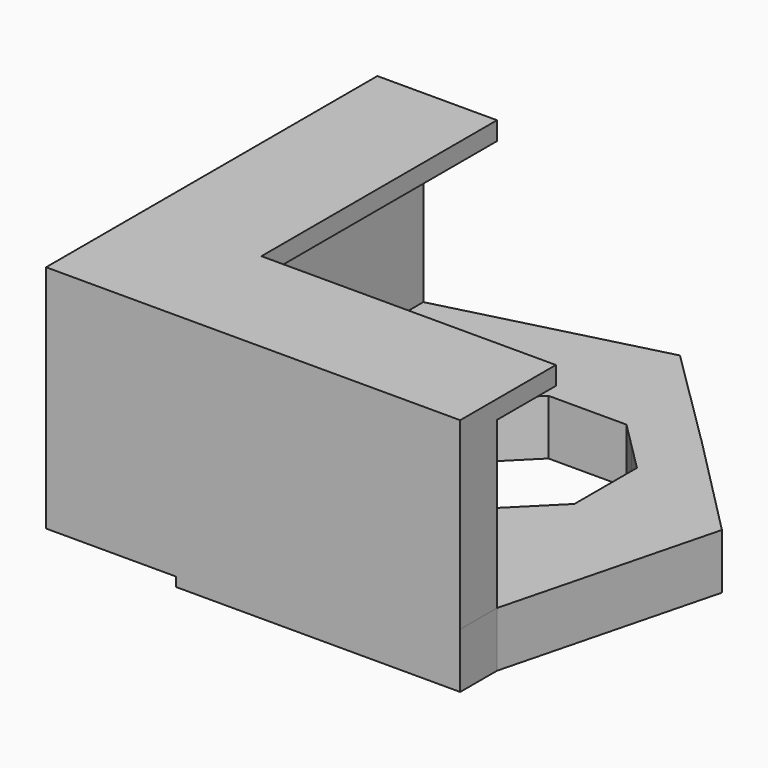
from build123d import *

# Parameters (mm, degrees)
F2_DEPTH  = 6
F4_DEPTH  = 3
F5_DEPTH  = 6.5
F7_DEPTH  = 1.5
F8_R      = 0.99999
F10_DEPTH = 1


# Not quite as in the source:
# - a fillet or chamfer is up to 0.001 mm smaller than in the source, because OpenCascade refuses the exact size


with BuildPart() as f2:
    # F1 (on offset) → F2 (new body)
    with BuildSketch(Plane.XY.offset(4)):
        Polygon((20, 0), (0, 0), (0, 20), (-2.5, 20), (-2.5, -2.5), (20, -2.5), align=None)
    extrude(amount=F2_DEPTH)



with BuildPart() as f4:
    # F3 (on Top) → F4 (new body)
    with BuildSketch(Plane.XY):
        Polygon((16.591883092, 13.7634559673), (16.591883092, 9.5208152802), (4.5710678119, -2.5), (8.75, -2.5), (22.9713253162, 11.5625), (17.2989898732, 17.2989898732), (15.1776695297, 15.1776695297), align=None)
        Polygon((22.9713253162, 11.5625), (8.75, -2.5), (20, -2.5), (20.0004931539, 0), align=None)
        Polygon((13.7634559673, 16.591883092), (15.1776695297, 15.1776695297), (17.2989898732, 17.2989898732), (11.5625, 22.9713253162), (-2.5, 8.75), (-2.5, 4.5710678119), (9.5208152802, 16.591883092), align=None)
        Polygon((-2.5, 8.75), (11.5625, 22.9713253162), (0, 19.9992582202), (-2.5, 20), align=None)
    extrude(amount=-F4_DEPTH)


with BuildPart() as f2_1:
    add(f2.part)

    add(f4.part)  # F5 merges F4
    # F1 (on offset) → F5 (join)
    with BuildSketch(Plane.XY.offset(4)):
        Polygon((20, 0), (0, 0), (0, 20), (-2.5, 20), (-2.5, -2.5), (20, -2.5), align=None)
    extrude(amount=-F5_DEPTH)

    # F6 (on face) → F7 (join)
    with BuildSketch(Plane(origin=(15.1776695297, 15.1776695297, 0), x_dir=(0.7071067812, -0.7071067812, 0), z_dir=(-0.7071067812, -0.7071067812, 0))):
        with BuildLine():
            Line((-1, -3), (1, -3))
            ThreePointArc((1, -3), (0, -2), (-1, -3))
        make_face()
    extrude(amount=F7_DEPTH)

    # F8 (radius 1 in the source; OpenCascade refuses exactly that, so slightly less here)
    f8_edges = [f2_1.edges().sort_by_distance(p)[0] for p in [
        (14.117009, 14.117009, -2),
    ]]
    fillet(f8_edges, radius=F8_R)

    # F9 (on face) → F10 (join)
    with BuildSketch(Plane.XY.offset(10)):
        Polygon((4, 20), (-2.5, 20), (-2.5, -2.5), (20, -2.5), (20, 4), (4, 4), align=None)
    extrude(amount=-F10_DEPTH)


solid = f2_1.part
